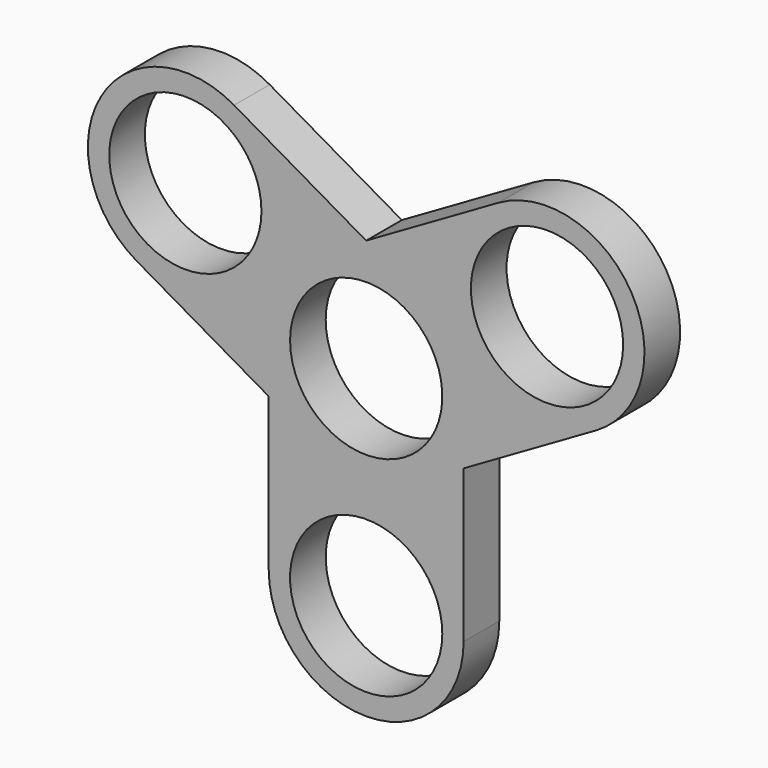
from build123d import *

# Parameters (mm, degrees)
F1_DEPTH        = 6.4
F1_COPIES_COUNT = 3


# Not quite as in the source:
# - a feature of the source that left no trace in its solid (it failed there, or was rolled back) is left out
# - a pattern or mirror of a feature is missing from the dataset's text; its kind, count and spacing are read off the source's solid


with BuildPart() as f1:
    # F0 (on Front) → F1 (new body)
    with BuildSketch(Plane.XZ):
        with BuildLine():
            Line((10.9347, -15), (14, -15))
            ThreePointArc((14, -15), (0, -1), (-14, -15))
            Line((-14, -15), (-10.9347, -15))
            ThreePointArc((-10.9347, -15), (0, -4.0653), (10.9347, -15))
        make_face()
        with BuildLine():
            ThreePointArc((-14, -15), (0, -29), (14, -15))
            Line((14, -15), (10.9347, -15))
            ThreePointArc((10.9347, -15), (0, -25.9347), (-10.9347, -15))
            Line((-10.9347, -15), (-14, -15))
        make_face()
        with BuildLine():
            ThreePointArc((-14, -15), (0, -1), (14, -15))
            Line((14, -15), (14, 15))
            ThreePointArc((14, 15), (0, 1), (-14, 15))
            Line((-14, 15), (-14, -15))
        make_face()
        with BuildLine():
            ThreePointArc((-14, 15), (0, 1), (14, 15))
            Line((14, 15), (10.9347, 15))
            ThreePointArc((10.9347, 15), (0, 4.0653), (-10.9347, 15))
            Line((-10.9347, 15), (-14, 15))
        make_face()
        with BuildLine():
            Line((10.9347, 15), (14, 15))
            ThreePointArc((14, 15), (0, 29), (-14, 15))
            Line((-14, 15), (-10.9347, 15))
            ThreePointArc((-10.9347, 15), (0, 25.9347), (10.9347, 15))
        make_face()
    extrude(amount=F1_DEPTH)

    # F1_copies: F1 ×3 about axis
    f1_copies_axis = Axis((0, 0, 15), (0, 1, 0))


with BuildPart() as f1_1:
    add(f1.part)
    for i in range(1, F1_COPIES_COUNT):
        add(f1.part.rotate(f1_copies_axis, i * 360 / F1_COPIES_COUNT))


solid = f1_1.part
